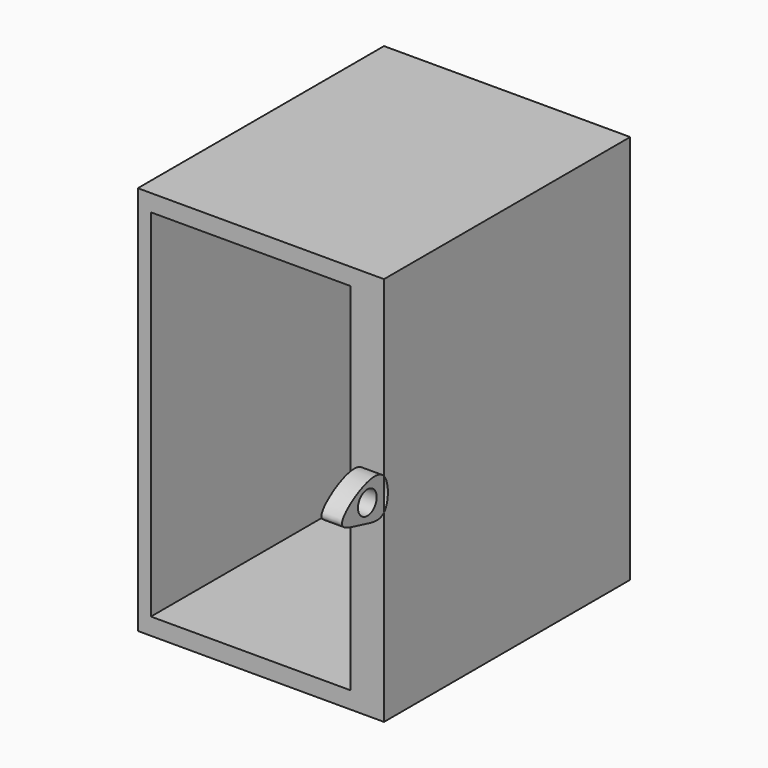
from build123d import *

# Parameters (mm, degrees)
F0_W     = 279.4
F0_H     = 482.6
F0_W_2   = 246.8713670969
F0_H_2   = 440.6119585037
F1_DEPTH = 381
F2_DEPTH = 25.4
F3_R     = 14.505640819
F4_DEPTH = 25.4


with BuildPart() as f1:
    # F0 (on Front) → F1 (new body)
    with BuildSketch(Plane.XZ):
        Rectangle(F0_W, F0_H)
        Rectangle(F0_W_2, F0_H_2, mode=Mode.SUBTRACT)
    extrude(amount=F1_DEPTH)

    # F0 (on Front) → F2 (join)
    with BuildSketch(Plane.XZ):
        Rectangle(F0_W_2, F0_H_2)
    extrude(amount=F2_DEPTH)

    # F3 (on face) → F4 (join)
    with BuildSketch(Plane.YZ.offset(139.7)):
        with BuildLine():
            Line((-381, -13.0550665781), (-381, 26.5936553478))
            add(Edge.make_bspline(
                [(-381, 26.5936553478), (-389.2777418759, 36.0344145926), (-422.144810442, 29.1111932624), (-459.0503806055, -3.6870125897), (-415.8766281026, -11.1937380865), (-388.4597489706, -20.8454898508), (-381, -13.0550665781)],
                knots=[0, 0, 0, 0, 0.2107256672, 0.4064612968, 0.5915610408, 0.7912039011, 0.7912039011, 0.7912039011, 0.7912039011], degree=3))
        make_face()
        with Locations((-406.7702889442, 8.2198567688)):
            Circle(F3_R, mode=Mode.SUBTRACT)
        with BuildLine():
            Line((-381, 241.3), (-381, 26.5936553478))
            add(Edge.make_bspline(
                [(-381, -13.0550665781), (-373.1982359839, -4.9074674835), (-372.7980555741, 17.2393430457), (-381, 26.5936553478)],
                knots=[0.7912039011, 0.7912039011, 0.7912039011, 0.7912039011, 1, 1, 1, 1], degree=3))
            Line((-381, -13.0550665781), (-381, -241.3))
            Line((-381, -241.3), (0, -241.3))
            Line((0, -241.3), (0, 241.3))
            Line((0, 241.3), (-381, 241.3))
        make_face()
    extrude(amount=F4_DEPTH)


solid = f1.part
